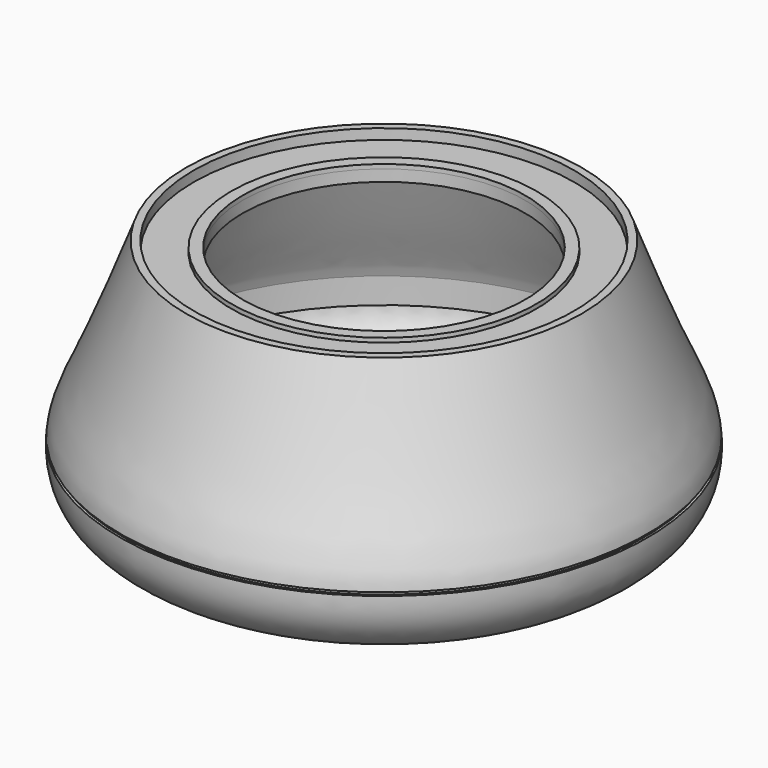
from build123d import *

# Parameters (mm, degrees)
F3_DEPTH        = 2
F3_COPIES_COUNT = 4
F4_T            = 2.5


# Not quite as in the source:
# - a pattern or mirror of a feature is missing from the dataset's text; its kind, count and spacing are read off the source's solid
# - a shell that OpenCascade refuses in one call is made with other operations: the cavity is built on its own and cut out


with BuildPart() as f1:
    # F0 (on Front) → F1 (revolve)
    with BuildSketch(Plane.XZ):
        with BuildLine():
            Line((-43.3527082205, 0), (0, 0))
            Line((0, 0), (0, 53.0404113233))
            Line((0, 53.0404113233), (-33.4537662566, 53.0404113233))
            Line((-33.4537662566, 53.0404113233), (-33.4537662566, 52.0980209112))
            Line((-33.4537662566, 52.0980209112), (-41.6996814311, 52.0980209112))
            Line((-41.6996814311, 52.0980209112), (-41.6996814311, 54.3659478426))
            Line((-41.6996814311, 54.3659478426), (-43.3527082205, 54.3659478426))
            add(Edge.make_bspline(
                [(-57.774114346, 16.6056844133), (-57.5438064684, 19.0766188083), (-55.1127232743, 26.0286261422), (-51.9674220523, 31.2399392322), (-43.3527082205, 54.3659478426)],
                knots=[0.378877356, 0.378877356, 0.378877356, 0.378877356, 0.5599059311, 1, 1, 1, 1], degree=3))
            Line((-57.774114346, 16.6056844133), (-57.301864028, 16.6056844133))
            Line((-57.301864028, 16.6056844133), (-57.301864028, 15.9044522338))
            Line((-57.301864028, 15.9044522338), (-57.825628846, 15.9044522338))
            add(Edge.make_bspline(
                [(-43.3527082205, 0), (-56.0080710607, 3.3208582414), (-58.0263130937, 10.5001905359), (-57.8371183322, 15.6912182455), (-57.825628846, 15.9044522338)],
                knots=[0, 0, 0, 0, 0.3469393009, 0.3620402142, 0.3620402142, 0.3620402142, 0.3620402142], degree=3))
        make_face()
    revolve(axis=Axis((0, 0, 26.5202056617), (0, 0, -1)))

    # F2 (on face) → F3 (join)
    with BuildSketch(Plane(origin=(0, 0, 0), x_dir=(1, 0, 0), z_dir=(0, 0, -1))):
        with BuildLine():
            ThreePointArc((-28.2869943814, 28.2869943814), (-28.2869943814, 24.0443536943), (-24.0443536943, 24.0443536943))
            Line((-24.0443536943, 24.0443536943), (-28.2869943814, 28.2869943814))
        make_face()
        with BuildLine():
            Line((-28.2869943814, 28.2869943814), (-24.0443536943, 24.0443536943))
            ThreePointArc((-24.0443536943, 24.0443536943), (-23.3940354403, 25.0176237408), (-23.1656740379, 26.1656740379))
            ThreePointArc((-23.1656740379, 26.1656740379), (-25.0176237408, 28.9373126354), (-28.2869943814, 28.2869943814))
        make_face()
    f3 = extrude(amount=F3_DEPTH)

    # F3_copies: F3 ×4 about axis
    f3_copies_axis = Axis((0, 0, 0), (0, 0, 1))
    for i in range(1, F3_COPIES_COUNT):
        add(f3.rotate(f3_copies_axis, i * 360 / F3_COPIES_COUNT))

    # F4: shell of thickness 2.5, made by hand


with BuildPart() as f4_core1:
    # F4_t2: copy of F1
    add(f1.part)

    # the walls: a layer under each face that stays
    f4_faces = [f4_core1.faces().sort_by_distance(p)[0] for p in [
        (-50.5523500528, -27.8171661666, 16.6056844133),
        (54.1679502624, 0, 27.3038486835),
        (57.301864028, 0, 16.2550683235),
        (-40.4625276724, -11.5607221921, 54.3659478426),
        (50.5974252403, -27.8419694444, 15.9044522338),
        (41.6996814311, 0, 53.2319843769),
        (55.6407613411, 0, 7.3399005986),
        (-27.7997876207, -27.7997876207, 52.0980209112),
        (0, 0, 0),
        (33.4537662566, 0, 52.5692161173),
        (28.2869943814, -28.2869943814, -1),
        (-28.2869943814, -28.2869943814, -1),
        (28.2869943814, 28.2869943814, -1),
        (-28.2869943814, 28.2869943814, -1),
        (26.1656740379, -26.1656740379, -2),
        (-26.1656740379, -26.1656740379, -2),
        (26.1656740379, 26.1656740379, -2),
        (-26.1656740379, 26.1656740379, -2),
    ]]
    thicken(f4_faces, amount=-F4_T, mode=Mode.SUBTRACT)

    # F4_s3 → F4_t4 (revolve, cut)
    with BuildSketch(Plane.XZ):
        Polygon((-57.326864028, 16.5806844133), (-57.301864028, 19.1056844133), (-54.801864028, 19.1056844133), (-54.801864028, 16.6056844133), align=None)
    revolve(axis=Axis((0, 0, 16.6056844133), (0, 0, -1)), mode=Mode.SUBTRACT)

    # F4_s5 → F4_t6 (revolve, cut)
    with BuildSketch(Plane.XZ):
        Polygon((-57.326864028, 15.9294522338), (-54.801864028, 15.9044522338), (-54.801864028, 13.4044522338), (-57.301864028, 13.4044522338), align=None)
    revolve(axis=Axis((0, 0, 15.9044522338), (0, 0, -1)), mode=Mode.SUBTRACT)

    # F4_s7 → F4_t8 (revolve, cut)
    with BuildSketch(Plane.XZ):
        Polygon((-41.6746814311, 52.1230209112), (-44.1996814311, 52.0980209112), (-44.1996814311, 49.5980209112), (-41.6996814311, 49.5980209112), align=None)
    revolve(axis=Axis((0, 0, 52.0980209112), (0, 0, -1)), mode=Mode.SUBTRACT)

    # F4_s9 → F4_t10 (revolve, cut)
    with BuildSketch(Plane.XZ):
        Polygon((-33.4787662566, 52.1230209112), (-33.4537662566, 49.5980209112), (-30.9537662566, 49.5980209112), (-30.9537662566, 52.0980209112), align=None)
    revolve(axis=Axis((0, 0, 52.0980209112), (0, 0, -1)), mode=Mode.SUBTRACT)

    # F4_s11 → F4_t12 (revolve, cut)
    with BuildSketch(Plane(origin=(0, 0, 0), x_dir=(0, 0, 1), z_dir=(-0.7071067812, -0.7071067812, 0))):
        Polygon((-0.025, -33.978851093), (2.5, -34.003851093), (2.5, -36.503851093), (0, -36.503851093), align=None)
    revolve(axis=Axis((26.1656740379, -26.1656740379, 0), (0, 0, -1)), mode=Mode.SUBTRACT)

    # F4_s13 → F4_t14 (revolve, cut)
    with BuildSketch(Plane(origin=(0, 0, 0), x_dir=(0, 0, 1), z_dir=(-0.7071067812, 0.7071067812, 0))):
        Polygon((-0.025, -33.978851093), (2.5, -34.003851093), (2.5, -36.503851093), (0, -36.503851093), align=None)
    revolve(axis=Axis((-26.1656740379, -26.1656740379, 0), (0, 0, -1)), mode=Mode.SUBTRACT)

    # F4_s15 → F4_t16 (revolve, cut)
    with BuildSketch(Plane(origin=(0, 0, 0), x_dir=(0, 0, 1), z_dir=(0.7071067812, -0.7071067812, 0))):
        Polygon((-0.025, -33.978851093), (2.5, -34.003851093), (2.5, -36.503851093), (0, -36.503851093), align=None)
    revolve(axis=Axis((26.1656740379, 26.1656740379, 0), (0, 0, -1)), mode=Mode.SUBTRACT)

    # F4_s17 → F4_t18 (revolve, cut)
    with BuildSketch(Plane(origin=(0, 0, 0), x_dir=(0, 0, 1), z_dir=(0.7071067812, 0.7071067812, 0))):
        Polygon((-0.025, -33.978851093), (2.5, -34.003851093), (2.5, -36.503851093), (0, -36.503851093), align=None)
    revolve(axis=Axis((-26.1656740379, 26.1656740379, 0), (0, 0, -1)), mode=Mode.SUBTRACT)


with BuildPart() as f1_1:
    add(f1.part)

    # what is left inside the walls is the cavity
    f4_cavity = [f4_core1.part.solids().sort_by_distance(p)[0] for p in [
        (52.796181, 0, 24.191952),
    ]]
    add(f4_cavity, mode=Mode.SUBTRACT)


solid = f1_1.part
